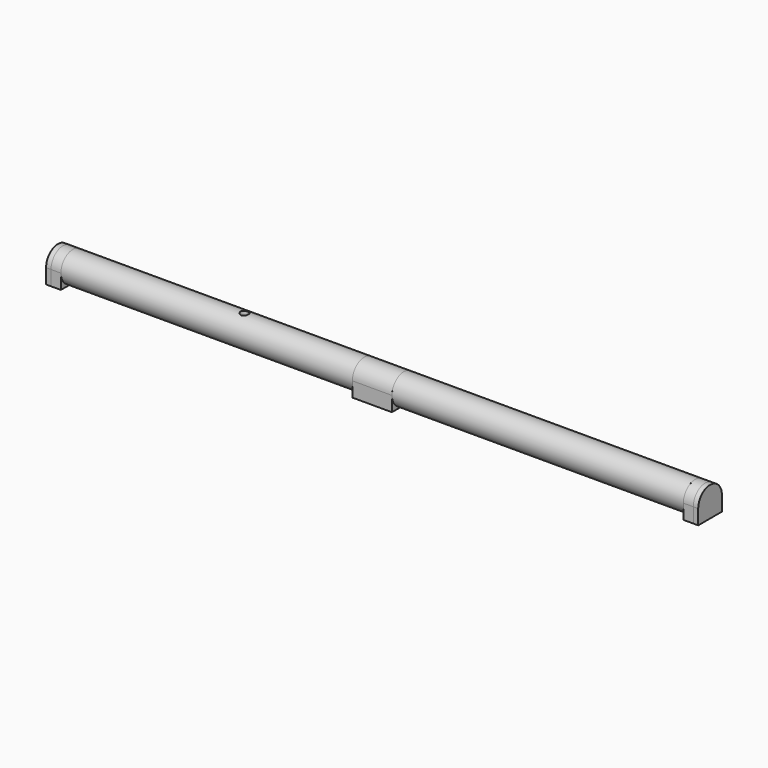
from build123d import *

# Parameters (mm, degrees)
F2_START       = 10
F1_R           = 7.5
F2_DEPTH       = 147.5
F4_D           = 10
F4_DEPTH       = 150
F4_TIP         = 3.0043030951
F0_R           = 5
F5_DEPTH       = 80
F5_DEPTH_BACK  = 80
F6_DEPTH       = 82.5
F7_START       = -10
F7_DEPTH       = 147.5
F9_D           = 10
F9_DEPTH       = 157.5
F9_TIP         = 3.0043030951
F10_DEPTH      = 82.5
F12_D          = 4
F12_DEPTH      = 90
F12_TIP        = 1.2017212381
F14_DEPTH      = 25
F16_DEPTH      = 5
F17_W          = 4
F17_H          = 1
F18_DEPTH      = 10
F19_R          = 2
F20_DEPTH      = 10
F22_START      = -157.5
F22_DEPTH      = 5
F23_START      = 157.5
F23_DEPTH      = 5
F24_DEPTH      = 10
F24_DEPTH_BACK = 10
F25_DEPTH      = 25
F27_START      = 162.5
F27_DEPTH      = 2.5
F28_START      = -162.5
F28_DEPTH      = 2.5


with BuildPart() as f2:
    # F1 (on Right) → F2 (new body)
    with BuildSketch(Plane.YZ.offset(F2_START)):
        Circle(F1_R)
    extrude(amount=F2_DEPTH)

    # F4
    with Locations(Plane.YZ.offset(157.5)):
        with Locations((0, 0)):
            Hole(F4_D / 2, depth=F4_DEPTH)
            with Locations((0, 0, -(F4_DEPTH + F4_TIP / 2))):  # 118° drill point
                Cone(0, F4_D / 2, F4_TIP, mode=Mode.SUBTRACT)


with BuildPart() as f5:
    # F0 (on Right) → F5 (new body, two sides)
    with BuildSketch(Plane.YZ) as f5_sk:
        Circle(F0_R)
    extrude(amount=F5_DEPTH)
    extrude(f5_sk.sketch, amount=-F5_DEPTH_BACK)


with BuildPart() as f6:
    # F6 (new): a face of the model
    f6_faces = [f5.part.faces().sort_by_distance(p)[0] for p in [
        (80, 0, 0),
    ]]
    extrude(f6_faces, amount=F6_DEPTH)


with BuildPart() as f7:
    # F1 (on Right) → F7 (new body)
    with BuildSketch(Plane.YZ.offset(F7_START)):
        Circle(F1_R)
    extrude(amount=-F7_DEPTH)

    # F9
    with Locations(Plane(origin=(-157.5, 0, 0), x_dir=(0, -1, 0), z_dir=(-1, 0, 0))):
        with Locations((0, 0)):
            Hole(F9_D / 2, depth=F9_DEPTH)
            with Locations((0, 0, -(F9_DEPTH + F9_TIP / 2))):  # 118° drill point
                Cone(0, F9_D / 2, F9_TIP, mode=Mode.SUBTRACT)

    # F19 (on Top) → F20 (cut)
    with BuildSketch(Plane.XY):
        with Locations((-70.56, 0)):
            Circle(F19_R)
    extrude(amount=F20_DEPTH, mode=Mode.SUBTRACT)


with BuildPart() as f10:
    # F10 (new): a face of the model
    f10_faces = [f5.part.faces().sort_by_distance(p)[0] for p in [
        (-80, 0, 0),
    ]]
    extrude(f10_faces, amount=F10_DEPTH)


with BuildPart() as f5_1:
    add(f5.part)

    # F12
    with Locations(Plane(origin=(-80, 0, 0), x_dir=(0, -1, 0), z_dir=(-1, 0, 0))):
        with Locations((0, 0)):
            Hole(F12_D / 2, depth=F12_DEPTH)
            with Locations((0, 0, -(F12_DEPTH + F12_TIP / 2))):  # 118° drill point
                Cone(0, F12_D / 2, F12_TIP, mode=Mode.SUBTRACT)

    # F13 (on Top) → F14 (cut)
    with BuildSketch(Plane.XY):
        with BuildLine():
            Line((-70.5600346923, 0.4569037808), (-70.5600346923, -0.0430962192))
            Line((-70.5600346923, -0.0430962192), (-68.5600346923, -0.0430962192))
            ThreePointArc((-68.5600346923, -0.0430962192), (-68.5759752998, 0.2089123658), (-68.6235430192, 0.4569037808))
            Line((-68.6235430192, 0.4569037808), (-70.5600346923, 0.4569037808))
        make_face()
        Polygon((-68.5600346923, -0.0430962192), (-70.5600346923, -0.0430962192), (-72.5600346923, -0.0430962192), (-72.5600346923, -5.0430962192), (-68.5600346923, -5.0430962192), align=None)
        with BuildLine():
            Line((-72.5600346923, -0.0430962192), (-70.5600346923, -0.0430962192))
            Line((-70.5600346923, -0.0430962192), (-70.5600346923, 0.4569037808))
            Line((-70.5600346923, 0.4569037808), (-72.4965263654, 0.4569037808))
            ThreePointArc((-72.4965263654, 0.4569037808), (-72.5440940848, 0.2089123658), (-72.5600346923, -0.0430962192))
        make_face()
        with BuildLine():
            Line((-72.4965263654, 0.4569037808), (-70.5600346923, 0.4569037808))
            Line((-70.5600346923, 0.4569037808), (-68.6235430192, 0.4569037808))
            ThreePointArc((-68.6235430192, 0.4569037808), (-70.5600346923, 1.9569037808), (-72.4965263654, 0.4569037808))
        make_face()
    extrude(amount=F14_DEPTH, mode=Mode.SUBTRACT)

    # F15 (on Front) → F16 (cut)
    with BuildSketch(Plane.XZ):
        Polygon((-72.56, 1), (-72.56, 0), (-72.56, -0.1), (-70.56, -0.1), (-68.56, -0.1), (-68.56, 0), (-68.56, 1), align=None)
        with BuildLine():
            Line((-70.56, -0.1), (-72.56, -0.1))
            ThreePointArc((-72.56, -0.1), (-70.56, -2.1), (-68.56, -0.1))
            Line((-68.56, -0.1), (-70.56, -0.1))
        make_face()
    extrude(amount=F16_DEPTH, mode=Mode.SUBTRACT)

    # F17 (on Top) → F18 (cut)
    with BuildSketch(Plane.XY):
        Rectangle(F17_W, F17_H)
        with BuildLine():
            Line((-2, 0.5), (2, 0.5))
            ThreePointArc((2, 0.5), (0, 2.5), (-2, 0.5))
        make_face()
        with BuildLine():
            ThreePointArc((-2, -0.5), (0, -2.5), (2, -0.5))
            Line((2, -0.5), (-2, -0.5))
        make_face()
    extrude(amount=-F18_DEPTH, mode=Mode.SUBTRACT)


with BuildPart() as f22:
    # F21 (on Right) → F22 (new body)
    with BuildSketch(Plane.YZ.offset(F22_START)):
        with BuildLine():
            Line((7.5, 0), (5, 0))
            ThreePointArc((5, 0), (3.5355339059, -3.5355339059), (0, -5))
            Line((0, -5), (0, -7.5))
            ThreePointArc((0, -7.5), (5.3033008589, -5.3033008589), (7.5, 0))
        make_face()
        with BuildLine():
            ThreePointArc((-5, 0), (0, 5), (5, 0))
            Line((5, 0), (7.5, 0))
            ThreePointArc((7.5, 0), (0, 7.5), (-7.5, 0))
            Line((-7.5, 0), (-5, 0))
        make_face()
        with BuildLine():
            ThreePointArc((0, -5), (-3.5355339059, -3.5355339059), (-5, 0))
            Line((-5, 0), (-7.5, 0))
            ThreePointArc((-7.5, 0), (-5.3033008589, -5.3033008589), (0, -7.5))
            Line((0, -7.5), (0, -5))
        make_face()
        with BuildLine():
            Line((7.5, -7.5), (7.5, 0))
            ThreePointArc((7.5, 0), (5.3033008589, -5.3033008589), (0, -7.5))
            Line((0, -7.5), (7.5, -7.5))
        make_face()
        with BuildLine():
            ThreePointArc((0, -7.5), (-5.3033008589, -5.3033008589), (-7.5, 0))
            Line((-7.5, 0), (-7.5, -7.5))
            Line((-7.5, -7.5), (0, -7.5))
        make_face()
    extrude(amount=-F22_DEPTH)


with BuildPart() as f23:
    # F21 (on Right) → F23 (new body)
    with BuildSketch(Plane.YZ.offset(F23_START)):
        with BuildLine():
            Line((7.5, 0), (5, 0))
            ThreePointArc((5, 0), (3.5355339059, -3.5355339059), (0, -5))
            Line((0, -5), (0, -7.5))
            ThreePointArc((0, -7.5), (5.3033008589, -5.3033008589), (7.5, 0))
        make_face()
        with BuildLine():
            ThreePointArc((-5, 0), (0, 5), (5, 0))
            Line((5, 0), (7.5, 0))
            ThreePointArc((7.5, 0), (0, 7.5), (-7.5, 0))
            Line((-7.5, 0), (-5, 0))
        make_face()
        with BuildLine():
            ThreePointArc((0, -5), (-3.5355339059, -3.5355339059), (-5, 0))
            Line((-5, 0), (-7.5, 0))
            ThreePointArc((-7.5, 0), (-5.3033008589, -5.3033008589), (0, -7.5))
            Line((0, -7.5), (0, -5))
        make_face()
        with BuildLine():
            Line((7.5, -7.5), (7.5, 0))
            ThreePointArc((7.5, 0), (5.3033008589, -5.3033008589), (0, -7.5))
            Line((0, -7.5), (7.5, -7.5))
        make_face()
        with BuildLine():
            ThreePointArc((0, -7.5), (-5.3033008589, -5.3033008589), (-7.5, 0))
            Line((-7.5, 0), (-7.5, -7.5))
            Line((-7.5, -7.5), (0, -7.5))
        make_face()
    extrude(amount=F23_DEPTH)


with BuildPart() as f24:
    # F21 (on Right) → F24 (new body, two sides)
    with BuildSketch(Plane.YZ) as f24_sk:
        with BuildLine():
            Line((7.5, 0), (5, 0))
            ThreePointArc((5, 0), (3.5355339059, -3.5355339059), (0, -5))
            Line((0, -5), (0, -7.5))
            ThreePointArc((0, -7.5), (5.3033008589, -5.3033008589), (7.5, 0))
        make_face()
        with BuildLine():
            ThreePointArc((-5, 0), (0, 5), (5, 0))
            Line((5, 0), (7.5, 0))
            ThreePointArc((7.5, 0), (0, 7.5), (-7.5, 0))
            Line((-7.5, 0), (-5, 0))
        make_face()
        with BuildLine():
            ThreePointArc((0, -5), (-3.5355339059, -3.5355339059), (-5, 0))
            Line((-5, 0), (-7.5, 0))
            ThreePointArc((-7.5, 0), (-5.3033008589, -5.3033008589), (0, -7.5))
            Line((0, -7.5), (0, -5))
        make_face()
        with BuildLine():
            Line((7.5, -7.5), (7.5, 0))
            ThreePointArc((7.5, 0), (5.3033008589, -5.3033008589), (0, -7.5))
            Line((0, -7.5), (7.5, -7.5))
        make_face()
        with BuildLine():
            ThreePointArc((0, -7.5), (-5.3033008589, -5.3033008589), (-7.5, 0))
            Line((-7.5, 0), (-7.5, -7.5))
            Line((-7.5, -7.5), (0, -7.5))
        make_face()
    extrude(amount=F24_DEPTH)
    extrude(f24_sk.sketch, amount=-F24_DEPTH_BACK)

    # F17 (on Top) → F25 (cut)
    with BuildSketch(Plane.XY):
        Rectangle(F17_W, F17_H)
        with BuildLine():
            Line((-2, 0.5), (2, 0.5))
            ThreePointArc((2, 0.5), (0, 2.5), (-2, 0.5))
        make_face()
        with BuildLine():
            ThreePointArc((-2, -0.5), (0, -2.5), (2, -0.5))
            Line((2, -0.5), (-2, -0.5))
        make_face()
    extrude(amount=-F25_DEPTH, mode=Mode.SUBTRACT)


with BuildPart() as f27:
    # F26 (on Right) → F27 (new body)
    with BuildSketch(Plane.YZ.offset(F27_START)):
        Polygon((5, 0), (0, 0), (-5, 0), (-7.5, 0), (-7.5, -7.5), (7.5, -7.5), (7.5, 0), align=None)
        with BuildLine():
            Line((-5, 0), (0, 0))
            Line((0, 0), (5, 0))
            Line((5, 0), (7.5, 0))
            ThreePointArc((7.5, 0), (0, 7.5), (-7.5, 0))
            Line((-7.5, 0), (-5, 0))
        make_face()
    extrude(amount=F27_DEPTH)


with BuildPart() as f28:
    # F26 (on Right) → F28 (new body)
    with BuildSketch(Plane.YZ.offset(F28_START)):
        Polygon((5, 0), (0, 0), (-5, 0), (-7.5, 0), (-7.5, -7.5), (7.5, -7.5), (7.5, 0), align=None)
        with BuildLine():
            Line((-5, 0), (0, 0))
            Line((0, 0), (5, 0))
            Line((5, 0), (7.5, 0))
            ThreePointArc((7.5, 0), (0, 7.5), (-7.5, 0))
            Line((-7.5, 0), (-5, 0))
        make_face()
    extrude(amount=-F28_DEPTH)


solid = Compound([f2.part, f6.part, f7.part, f10.part, f5_1.part, f22.part, f23.part, f24.part, f27.part, f28.part])
